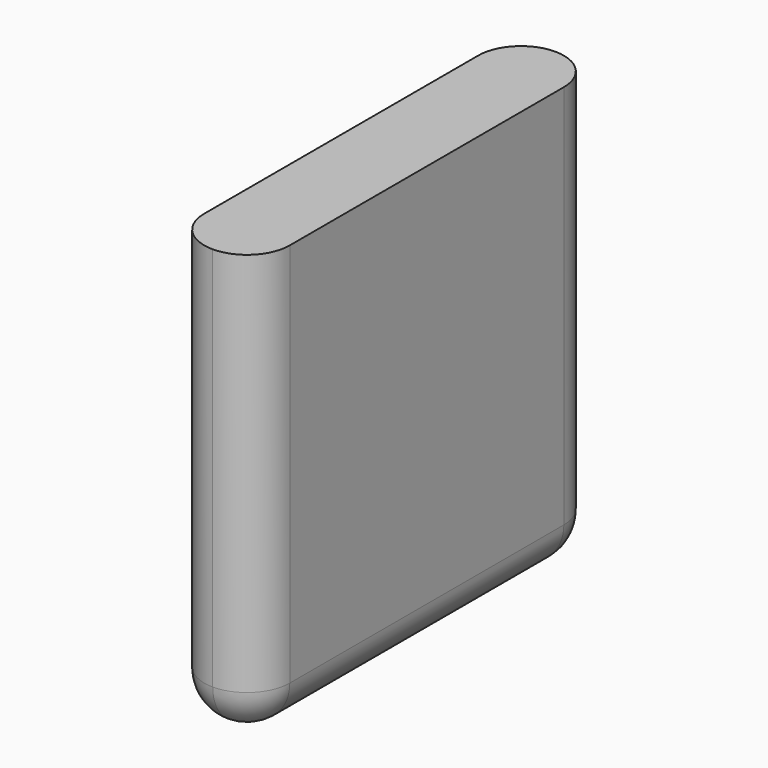
from build123d import *

# Parameters (mm, degrees)
F0_W     = 1
F0_H     = 5
F1_DEPTH = 5
F2_R     = 0.49999


# Not quite as in the source:
# - a fillet or chamfer is up to 0.001 mm smaller than in the source, because OpenCascade refuses the exact size


with BuildPart() as f1:
    # F0 (on Top) → F1 (new body)
    with BuildSketch(Plane.XY):
        Rectangle(F0_W, F0_H)
    extrude(amount=F1_DEPTH)

    # F2 (radius 0.5 in the source; OpenCascade refuses exactly that, so slightly less here)
    f2_edges = [f1.edges().sort_by_distance(p)[0] for p in [
        (0, 2.5, 0),
        (-0.5, 0, 0),
        (0, -2.5, 0),
        (0.5, 0, 0),
        (0.5, 2.5, 2.5),
        (-0.5, 2.5, 2.5),
        (-0.5, -2.5, 2.5),
        (0.5, -2.5, 2.5),
    ]]
    fillet(f2_edges, radius=F2_R)


solid = f1.part
